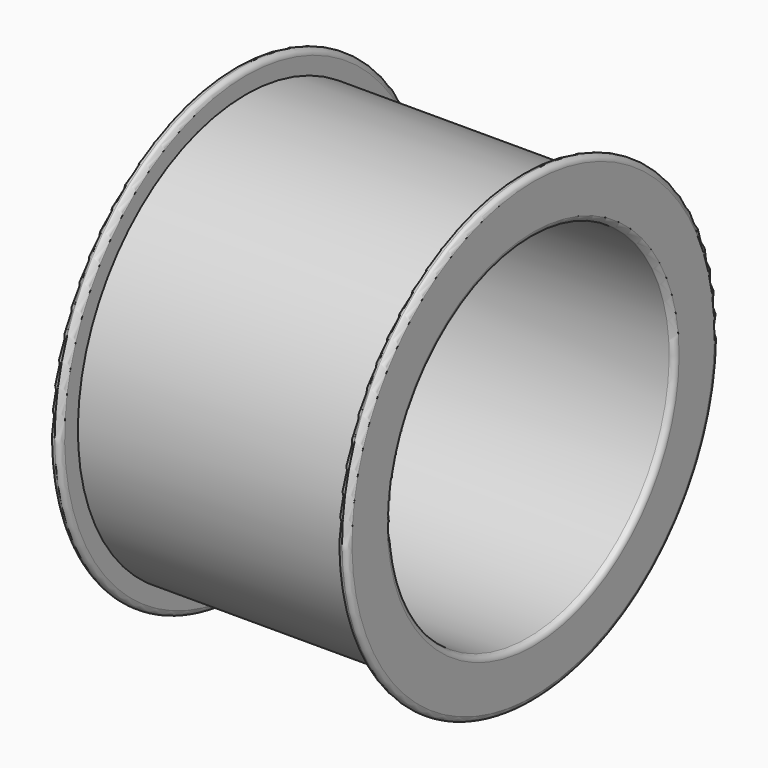
from build123d import *

# Parameters (mm, degrees)
F3_R = 0.49999
F4_R = 0.5


# Not quite as in the source:
# - a fillet or chamfer is up to 0.001 mm smaller than in the source, because OpenCascade refuses the exact size


with BuildPart() as f2:
    # F0 (on Front) → F2 (revolve)
    with BuildSketch(Plane.XZ):
        Polygon((-20.462457691, 21), (-20.462457691, 16), (6.537542309, 16), (6.537542309, 21), (5.537542309, 21), (5.537542309, 19), (-19.462457691, 19), (-19.462457691, 21), align=None)
    revolve(axis=Axis((-6.0107018799, 0, 0), (1, 0, 0)))

    # F3 (radius 0.5 in the source; OpenCascade refuses exactly that, so slightly less here)
    f3_edges = [f2.edges().sort_by_distance(p)[0] for p in [
        (6.537542, 0, -21),
        (5.537542, 0, -21),
        (-19.462458, 0, -21),
        (-20.462458, 0, -21),
    ]]
    fillet(f3_edges, radius=F3_R)

    # F4
    f4_edges = [f2.edges().sort_by_distance(p)[0] for p in [
        (-20.462458, 0, -16),
        (6.537542, 0, -16),
    ]]
    fillet(f4_edges, radius=F4_R)


solid = f2.part
